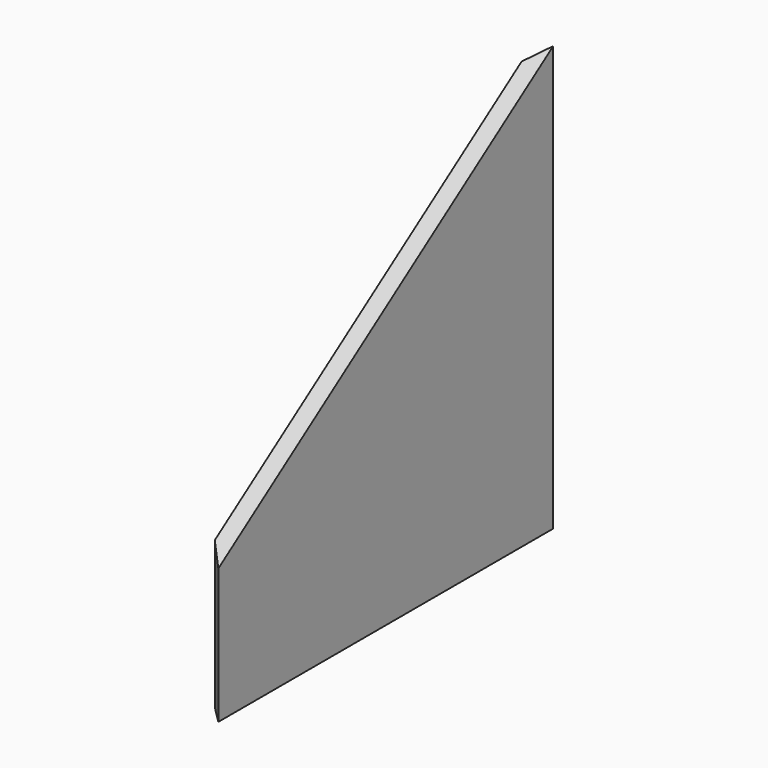
from build123d import *

# Parameters (mm, degrees)
F1_DEPTH    = 4.0000047
F2_T1_DEPTH = 112.2565983155
F3_T1_DEPTH = 247.2565983155


# Not quite as in the source:
# - a fillet or chamfer that OpenCascade refuses, or shapes differently, is made with other operations: its cross-section is extruded or revolved along the edge and cut away or added


with BuildPart() as f1:
    # F0 (on Right) → F1 (new body, symmetric)
    with BuildSketch(Plane.YZ):
        Polygon((-99.9751089393, -29.498891169), (-99.9751089393, -89.4988911689), (95.0248910607, -89.4988911689), (95.0248910607, 105.5011088311), align=None)
    extrude(amount=F1_DEPTH, both=True)

    # F2: chamfer of 10.16 on 1 edges, made by hand

    # F2_s2 → F2_t1 (cut)
    with BuildSketch(Plane.XY.offset(-115.6271903267)):
        Polygon((6.1599953, -99.9751089393), (-4.0000047, -89.8151089393), (-4.0000047, -99.9751089393), align=None)
    extrude(amount=F2_T1_DEPTH, mode=Mode.SUBTRACT)

    # F3: chamfer of 10.16 on 1 edges, made by hand

    # F3_s2 → F3_t1 (cut)
    with BuildSketch(Plane.XY.offset(-115.6271903267)):
        Polygon((-4.0000047, 84.8648910607), (6.1599953, 95.0248910607), (-4.0000047, 95.0248910607), align=None)
    extrude(amount=F3_T1_DEPTH, mode=Mode.SUBTRACT)


solid = f1.part
